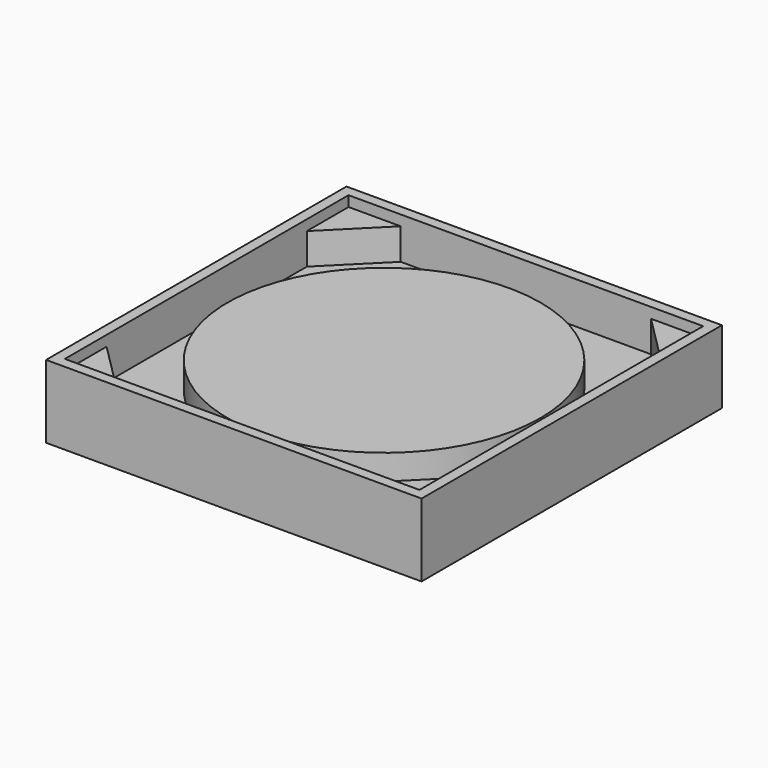
from build123d import *

# Parameters (mm, degrees)
F1_R      = 150
F2_DEPTH  = 35
F3_R      = 150
F4_DEPTH  = 10
F5_DEPTH  = 10
F6_W      = 360
F6_H      = 360
F7_DEPTH  = 10
F8_W      = 10
F8_H      = 340
F9_DEPTH  = 60
F11_DEPTH = 50


with BuildPart() as f2:
    # F1 (on Top) → F2 (new body)
    with BuildSketch(Plane.XY):
        Circle(F1_R)
    extrude(amount=F2_DEPTH)


with BuildPart() as f4:
    # F3 (on face) → F4 (new body)
    with BuildSketch(Plane(origin=(0, 0, 0), x_dir=(1, 0, 0), z_dir=(0, 0, -1))):
        Polygon((120, 170), (-120, 170), (-170, 120), (-170, -120), (-120, -170), (120, -170), (170, -120), (170, 120), align=None)
        Circle(F3_R, mode=Mode.SUBTRACT)
        Circle(F3_R)
    extrude(amount=F4_DEPTH)


with BuildPart() as f5:
    # F5 (new): a face of the model
    f5_faces = [f4.part.faces().sort_by_distance(p)[0] for p in [
        (0, 0, 0),
    ]]
    extrude(f5_faces, amount=F5_DEPTH)


with BuildPart() as f7:
    # F6 (on face) → F7 (new body)
    with BuildSketch(Plane(origin=(0, 0, -10), x_dir=(1, 0, 0), z_dir=(0, 0, -1))):
        Rectangle(F6_W, F6_H)
        Polygon((-120, 170), (120, 170), (170, 120), (170, -120), (120, -170), (-120, -170), (-170, -120), (-170, 120), align=None, mode=Mode.SUBTRACT)
        Polygon((170, 120), (120, 170), (-120, 170), (-170, 120), (-170, -120), (-120, -170), (120, -170), (170, -120), align=None)
    extrude(amount=F7_DEPTH)

    # F8 (on face) → F9 (join)
    with BuildSketch(Plane.XY.offset(-10)):
        Polygon((-180, -170), (-180, -180), (180, -180), (180, -170), (170, -170), (-170, -170), align=None)
        with Locations((-175, 0)):
            Rectangle(F8_W, F8_H)
        Polygon((-180, 180), (-180, 170), (-170, 170), (170, 170), (180, 170), (180, 180), align=None)
        with Locations((175, 0)):
            Rectangle(F8_W, F8_H)
    extrude(amount=F9_DEPTH)

    # F10 (on face) → F11 (join)
    with BuildSketch(Plane.XY.offset(-10)):
        Polygon((-170, -170), (-120, -170), (-170, -120), align=None)
        Polygon((120, -170), (170, -170), (170, -120), align=None)
        Polygon((120, 170), (170, 120), (170, 170), align=None)
        Polygon((-170, 170), (-170, 120), (-120, 170), align=None)
    extrude(amount=F11_DEPTH)


solid = Compound([f2.part, f4.part, f5.part, f7.part])
